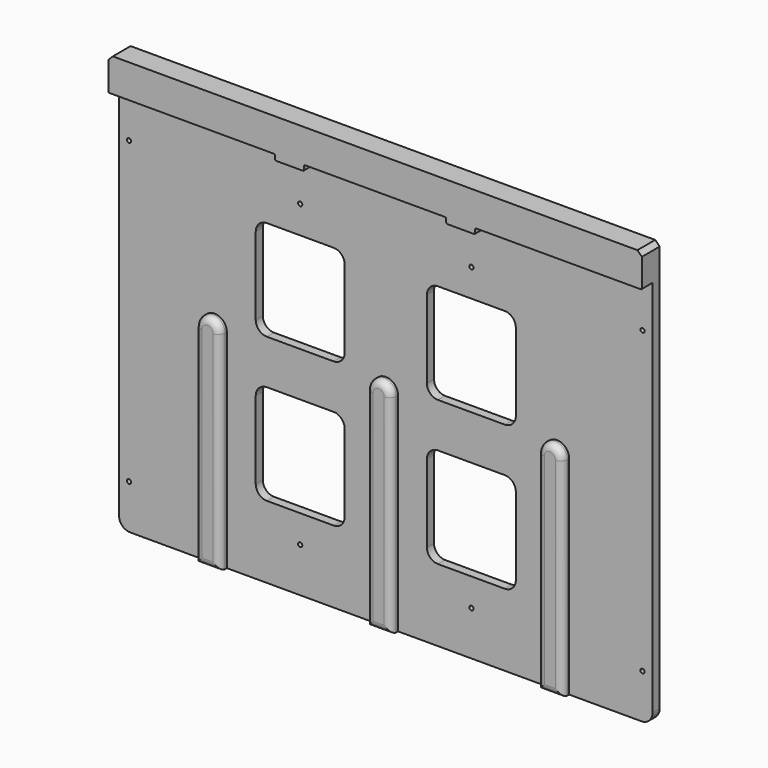
from build123d import *

# Parameters (mm, degrees)
F0_R     = 0.95
F0_W     = 40
F0_H     = 45
F0_W_2   = 75
F0_H_2   = 15
F0_W_3   = 64
F1_DEPTH = 4
F2_DEPTH = 8
F3_DEPTH = 10
F4_R     = 5
F5_SIZE  = 2
F6_R     = 3
F7_R     = 0.5


# Not quite as in the source:
# - a feature names something its author has since deleted; it is built from what else it names


with BuildPart() as f1:
    # F0 (on Front) → F1 (new body)
    with BuildSketch(Plane.XZ):
        with BuildLine():
            Line((0, 175), (0, 0))
            Line((0, 0), (37.5, 0))
            Line((37.5, 0), (37.5, 93.5))
            ThreePointArc((37.5, 93.5), (43, 99), (48.5, 93.5))
            Line((48.5, 93.5), (48.5, 0))
            Line((48.5, 0), (114.5, 0))
            Line((114.5, 0), (114.5, 93.5))
            ThreePointArc((114.5, 93.5), (120, 99), (125.5, 93.5))
            Line((125.5, 93.5), (125.5, 0))
            Line((125.5, 0), (191.5, 0))
            Line((191.5, 0), (191.5, 93.5))
            ThreePointArc((191.5, 93.5), (197, 99), (202.5, 93.5))
            Line((202.5, 93.5), (202.5, 0))
            Line((202.5, 0), (240, 0))
            Line((240, 0), (240, 175))
            Line((240, 175), (165, 175))
            Line((165, 175), (165, 172.5))
            Line((165, 172.5), (152, 172.5))
            Line((152, 172.5), (152, 175))
            Line((152, 175), (88, 175))
            Line((88, 175), (88, 172.5))
            Line((88, 172.5), (75, 172.5))
            Line((75, 172.5), (75, 175))
            Line((75, 175), (0, 175))
        make_face()
        with Locations((4.5, 20)):
            Circle(F0_R, mode=Mode.SUBTRACT)
        with Locations((81.5, 20)):
            Circle(F0_R, mode=Mode.SUBTRACT)
        with Locations((81.5, 55)):
            Rectangle(F0_W, F0_H, mode=Mode.SUBTRACT)
        with Locations((158.5, 20)):
            Circle(F0_R, mode=Mode.SUBTRACT)
        with Locations((235.5, 20)):
            Circle(F0_R, mode=Mode.SUBTRACT)
        with Locations((158.5, 55)):
            Rectangle(F0_W, F0_H, mode=Mode.SUBTRACT)
        with Locations((81.5, 120)):
            Rectangle(F0_W, F0_H, mode=Mode.SUBTRACT)
        with Locations((4.5, 155)):
            Circle(F0_R, mode=Mode.SUBTRACT)
        with Locations((81.5, 155)):
            Circle(F0_R, mode=Mode.SUBTRACT)
        with Locations((158.5, 120)):
            Rectangle(F0_W, F0_H, mode=Mode.SUBTRACT)
        with Locations((158.5, 155)):
            Circle(F0_R, mode=Mode.SUBTRACT)
        with Locations((235.5, 155)):
            Circle(F0_R, mode=Mode.SUBTRACT)
        with Locations((202.5, 182.5)):
            Rectangle(F0_W_2, F0_H_2)
        Polygon((165, 190), (152, 190), (152, 175), (152, 172.5), (165, 172.5), (165, 175), align=None)
        with Locations((120, 182.5)):
            Rectangle(F0_W_3, F0_H_2)
        Polygon((75, 190), (75, 175), (75, 172.5), (88, 172.5), (88, 175), (88, 190), align=None)
        with Locations((37.5, 182.5)):
            Rectangle(F0_W_2, F0_H_2)
        with BuildLine():
            Line((37.5, 93.5), (37.5, 0))
            Line((37.5, 0), (48.5, 0))
            Line((48.5, 0), (48.5, 93.5))
            ThreePointArc((48.5, 93.5), (43, 99), (37.5, 93.5))
        make_face()
        with BuildLine():
            Line((114.5, 93.5), (114.5, 0))
            Line((114.5, 0), (125.5, 0))
            Line((125.5, 0), (125.5, 93.5))
            ThreePointArc((125.5, 93.5), (120, 99), (114.5, 93.5))
        make_face()
        with BuildLine():
            Line((191.5, 93.5), (191.5, 0))
            Line((191.5, 0), (202.5, 0))
            Line((202.5, 0), (202.5, 93.5))
            ThreePointArc((202.5, 93.5), (197, 99), (191.5, 93.5))
        make_face()
    extrude(amount=F1_DEPTH)

    # F0 (on Front) → F2 (join)
    with BuildSketch(Plane.XZ):
        with BuildLine():
            Line((37.5, 93.5), (37.5, 0))
            Line((37.5, 0), (48.5, 0))
            Line((48.5, 0), (48.5, 93.5))
            ThreePointArc((48.5, 93.5), (43, 99), (37.5, 93.5))
        make_face()
        with BuildLine():
            Line((114.5, 93.5), (114.5, 0))
            Line((114.5, 0), (125.5, 0))
            Line((125.5, 0), (125.5, 93.5))
            ThreePointArc((125.5, 93.5), (120, 99), (114.5, 93.5))
        make_face()
        with BuildLine():
            Line((191.5, 93.5), (191.5, 0))
            Line((191.5, 0), (202.5, 0))
            Line((202.5, 0), (202.5, 93.5))
            ThreePointArc((202.5, 93.5), (197, 99), (191.5, 93.5))
        make_face()
    extrude(amount=F2_DEPTH)

    # F0 (on Front) → F3 (join)
    with BuildSketch(Plane.XZ):
        Polygon((75, 190), (75, 175), (75, 172.5), (88, 172.5), (88, 175), (88, 190), align=None)
        Polygon((165, 190), (152, 190), (152, 175), (152, 172.5), (165, 172.5), (165, 175), align=None)
        with Locations((202.5, 182.5)):
            Rectangle(F0_W_2, F0_H_2)
        with Locations((120, 182.5)):
            Rectangle(F0_W_3, F0_H_2)
        with Locations((37.5, 182.5)):
            Rectangle(F0_W_2, F0_H_2)
    extrude(amount=F3_DEPTH)

    # F4
    f4_edges = [f1.edges().sort_by_distance(p)[0] for p in [
        (0, -2, 0),
        (240, -2, 0),
        (138.5, -2, 32.5),
        (178.5, -2, 32.5),
        (178.5, -2, 77.5),
        (138.5, -2, 77.5),
        (138.5, -2, 142.5),
        (178.5, -2, 142.5),
        (178.5, -2, 97.5),
        (138.5, -2, 97.5),
        (61.5, -2, 32.5),
        (101.5, -2, 32.5),
        (101.5, -2, 77.5),
        (61.5, -2, 77.5),
        (101.5, -2, 97.5),
        (101.5, -2, 142.5),
        (61.5, -2, 142.5),
        (61.5, -2, 97.5),
    ]]
    fillet(f4_edges, radius=F4_R)

    # F5
    f5_edges = [f1.edges().sort_by_distance(p)[0] for p in [
        (240, -5, 190),
        (0, -5, 190),
    ]]
    chamfer(f5_edges, length=F5_SIZE)

    # F6
    f6_edges = [f1.edges().sort_by_distance(p)[0] for p in [
        (37.5, -8, 46.75),
        (43, -8, 0),
        (48.5, -8, 46.75),
        (43, -8, 99),
        (114.5, -8, 46.75),
        (120, -8, 0),
        (125.5, -8, 46.75),
        (120, -8, 99),
        (191.5, -8, 46.75),
        (197, -8, 0),
        (202.5, -8, 46.75),
        (197, -8, 99),
    ]]
    fillet(f6_edges, radius=F6_R)

    # F7
    f7_edges = [f1.edges().sort_by_distance(p)[0] for p in [
        (75, -7, 172.5),
        (75, -7, 175),
        (88, -7, 172.5),
        (88, -7, 175),
        (152, -7, 175),
        (152, -7, 172.5),
        (165, -7, 172.5),
        (165, -7, 175),
        (240, -7, 175),
        (0, -7, 175),
    ]]
    fillet(f7_edges, radius=F7_R)


solid = f1.part
